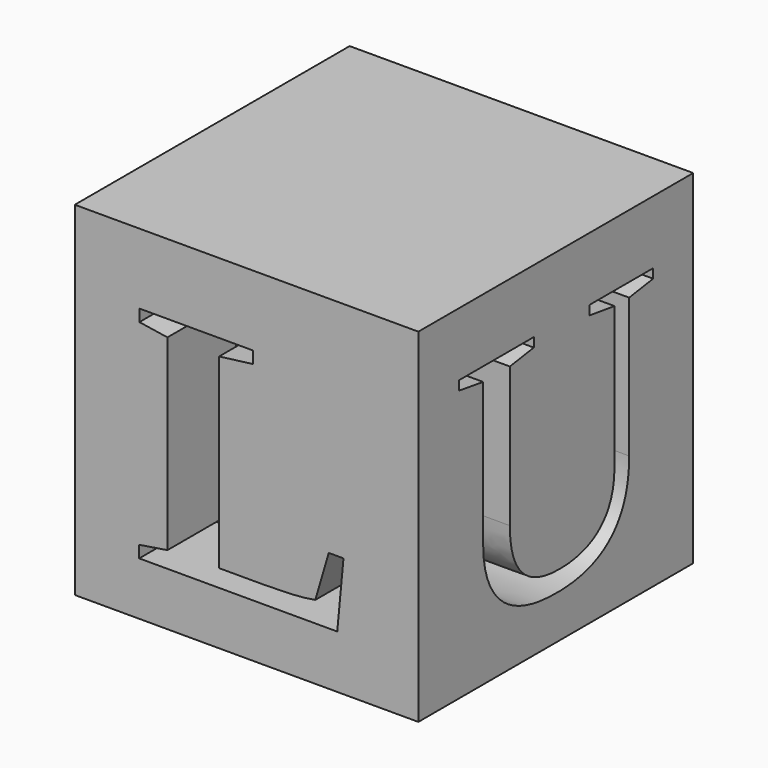
from build123d import *

# Parameters (mm, degrees)
F0_W         = 25.4
F0_H         = 25.4
F1_DEPTH     = 25.4
F2_TEXT_SIZE = 24.8403469515
F5_DEPTH     = 6.35
F4_TEXT_SIZE = 25.901316096
F6_DEPTH     = 6.35
F3_TEXT_SIZE = 26.3471660825
F7_DEPTH     = 6.35
F8_TEXT_SIZE = 25.901316096
F9_DEPTH     = 6.35


# Not quite as in the source:
# - Text() gives the source's letters only with a copy of the font that has no kerning and outlines rounded to 1/6400 em; it was checked with that copy


with BuildPart() as f1:
    # F0 (on Front) → F1 (new body)
    with BuildSketch(Plane.XZ):
        Rectangle(F0_W, F0_H)
    extrude(amount=F1_DEPTH)

    # F2 (on face) → F5 (cut)
    with BuildSketch(Plane.XZ.offset(25.4)):
        with Locations((-8.3606868284, -8.767683059)):
            Text('L', F2_TEXT_SIZE, font='Tinos', font_style=FontStyle.BOLD, text_align=(TextAlign.LEFT, TextAlign.BOTTOM))
    extrude(amount=-F5_DEPTH, mode=Mode.SUBTRACT)

    # F4 (on face) → F6 (cut)
    with BuildSketch(Plane(origin=(-12.7, 0, 0), x_dir=(0, -1, 0), z_dir=(-1, 0, 0))):
        with Locations((4.3942374177, -9.0956741769)):
            Text('E', F4_TEXT_SIZE, font='Tinos', text_align=(TextAlign.LEFT, TextAlign.BOTTOM))
    extrude(amount=-F6_DEPTH, mode=Mode.SUBTRACT)

    # F3 (on face) → F7 (cut)
    with BuildSketch(Plane.YZ.offset(12.7)):
        with Locations((-22.179541178, -9.2423260212)):
            Text('U', F3_TEXT_SIZE, font='Tinos', text_align=(TextAlign.LEFT, TextAlign.BOTTOM))
    extrude(amount=-F7_DEPTH, mode=Mode.SUBTRACT)

    # F8 (on face) → F9 (cut)
    with BuildSketch(Plane(origin=(0, 0, 0), x_dir=(-1, 0, 0), z_dir=(0, 1, 0))):
        with Locations((-10.0286658259, -9.4748679549)):
            Text('K', F8_TEXT_SIZE, font='Tinos', text_align=(TextAlign.LEFT, TextAlign.BOTTOM))
    extrude(amount=-F9_DEPTH, mode=Mode.SUBTRACT)


solid = f1.part
